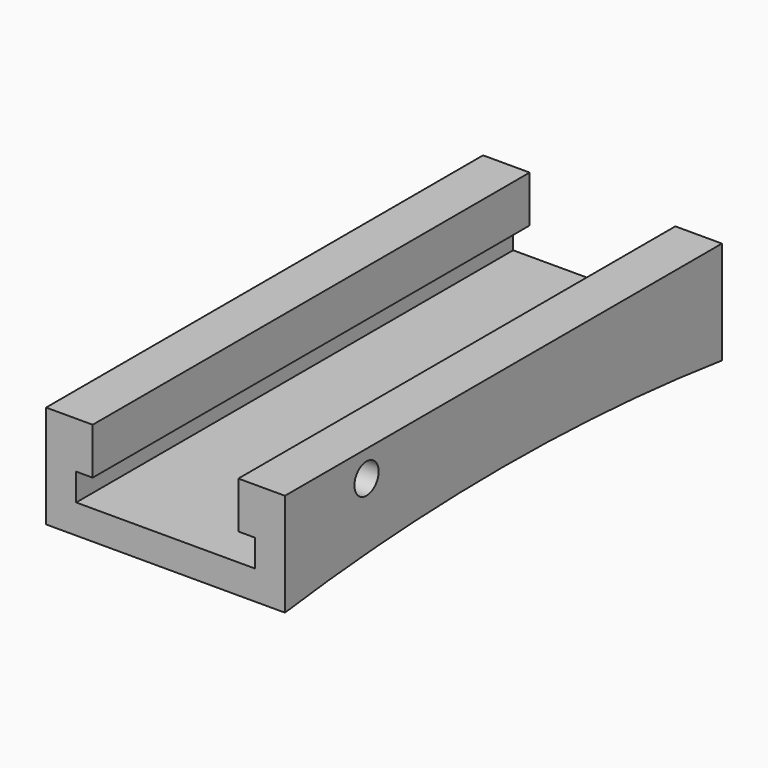
from build123d import *

# Parameters (mm, degrees)
F1_DEPTH = 71.4375
F2_R     = 1.9812
F3_DEPTH = 6.096
F5_DEPTH = 31.243


# Not quite as in the source:
# - a feature names something its author has since deleted; it is built from what else it names


with BuildPart() as f1:
    # F0 (on Front) → F1 (new body)
    with BuildSketch(Plane.XZ):
        Polygon((3.1813341729, 6.0924417882), (3.1813341729, 12.1884417882), (-2.9146658271, 12.1884417882), (-2.9146658271, -1.2735582118), (28.3273341729, -1.2735582118), (28.3273341729, 12.1884417882), (22.2313341729, 12.1884417882), (22.2313341729, 6.0924417882), (24.3903341729, 6.0924417882), (24.3903341729, 2.5364417882), (1.0223341729, 2.5364417882), (1.0223341729, 6.0924417882), align=None)
    extrude(amount=F1_DEPTH)

    # F2 (on face) → F3 (cut, through all)
    with BuildSketch(Plane.YZ.offset(28.3273341729)):
        with Locations((-58.1025, 8.7594417882)):
            Circle(F2_R)
    extrude(amount=-F3_DEPTH, mode=Mode.SUBTRACT)

    # F4 (on face) → F5 (cut, through all)
    with BuildSketch(Plane.YZ.offset(28.3273341729)):
        with BuildLine():
            ThreePointArc((0, -1.2735582118), (-35.71875, 1.0124417882), (-71.4375, -1.2735582118))
            Line((-71.4375, -1.2735582118), (0, -1.2735582118))
        make_face()
    extrude(amount=-F5_DEPTH, mode=Mode.SUBTRACT)


solid = f1.part
